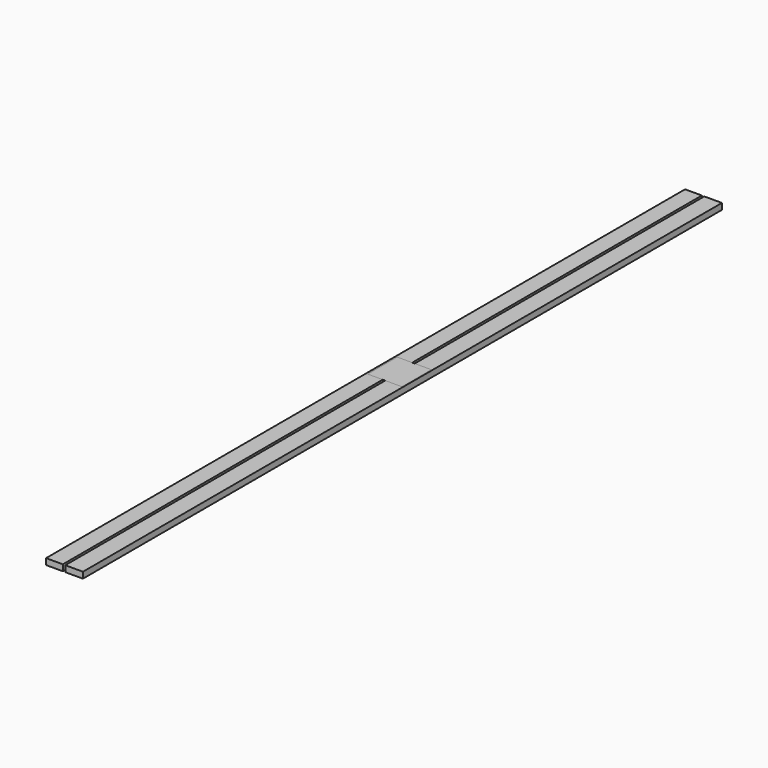
from build123d import *

# Parameters (mm, degrees)
F0_W     = 38.1
F0_H     = 825.5
F2_DEPTH = 6.35
F1_W     = 2.54
F1_H     = 990.6
F3_DEPTH = 284.48
F4_W     = 35.2549552917
F4_H     = 38.1
F5_DEPTH = 6.35


# Not quite as in the source:
# - a feature of the source that left no trace in its solid (it failed there, or was rolled back) is left out


with BuildPart() as f2:
    # F0 (on Top) → F2 (new body)
    with BuildSketch(Plane.XY):
        with Locations((-162.8751962613, -0.5595125258)):
            Rectangle(F0_W, F0_H)
    extrude(amount=F2_DEPTH)

    # F1 (on face) → F3 (cut)
    with BuildSketch(Plane.XY):
        with Locations((-163.3307448435, -60.3681156158)):
            Rectangle(F1_W, F1_H)
    extrude(amount=F3_DEPTH, mode=Mode.SUBTRACT)


with BuildPart() as f5:
    # F4 (on face) → F5 (new body)
    with BuildSketch(Plane.XY):
        with Locations((-162.5160872936, 19.05)):
            Rectangle(F4_W, F4_H)
    extrude(amount=F5_DEPTH)


solid = Compound([f2.part, f5.part])
